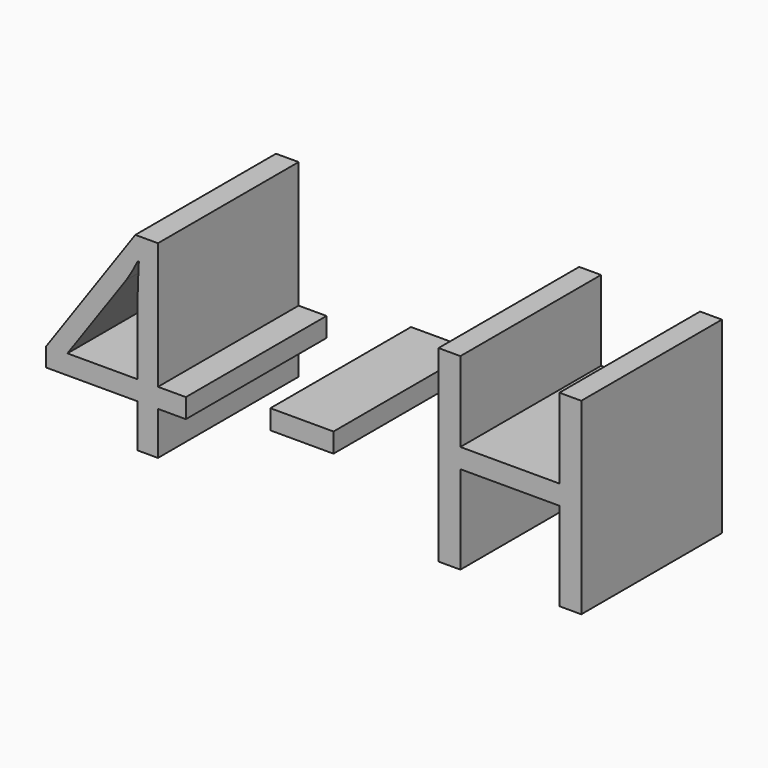
from build123d import *

# Parameters (mm, degrees)
F0_TEXT_SIZE = 38.0447315466
F1_DEPTH     = 25.4


# Not quite as in the source:
# - Text() gives the source's letters only with a copy of the font that has no kerning and outlines rounded to 1/6400 em; it was checked with that copy


with BuildPart() as f1:
    # F0 (on Front) → F1 (new body)
    with BuildSketch(Plane.XZ):
        with Locations((0, 0)):
            Text('4 - H', F0_TEXT_SIZE, font='Open Sans', text_align=(TextAlign.LEFT, TextAlign.BOTTOM))
    extrude(amount=F1_DEPTH)


solid = f1.part
